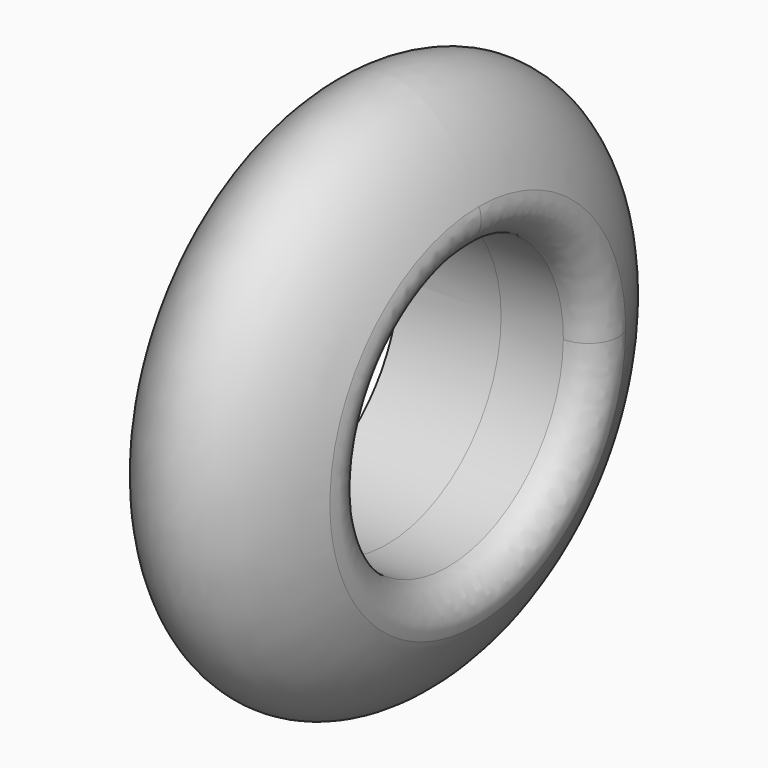
from build123d import *

# Parameters (mm, degrees)
F2_R     = 23.2302893252
F3_DEPTH = 18.4935515739
F4_R     = 20
F5_DEPTH = 18.8526750544
F6_R     = 5
F7_DEPTH = 17.3718996871


with BuildPart() as f1:
    # F0 (on Front) → F1 (revolve)
    with BuildSketch(Plane.XZ):
        with BuildLine():
            Line((-17.606544705, -0.1475060738), (17.5061281593, -0.703891208))
            add(Edge.make_bspline(
                [(17.5061281593, -0.703891208), (25.7537951553, 43.7031499409), (0.1598772489, 44.1087036708), (-25.4340406574, 44.5142574008), (-17.606544705, -0.1475060738)],
                knots=[4.3842952705, 4.3842952705, 4.3842952705, 6.2745397051, 6.2745397051, 8.1647841398, 8.1647841398, 8.1647841398], degree=2, weights=[1, 0.5856438179, 1, 0.5856438179, 1]))
        make_face()
    revolve(axis=Axis((-0.0502082729, 0, -0.4256986409), (0.9998744804, 0, -0.0158437183)))

    # F2 (on Right) → F3 (cut, through all)
    with BuildSketch(Plane.YZ):
        Circle(F2_R)
    extrude(amount=F3_DEPTH, mode=Mode.SUBTRACT)

    # F4 (on Right) → F5 (cut, through all)
    with BuildSketch(Plane.YZ):
        Circle(F4_R)
    extrude(amount=-F5_DEPTH, mode=Mode.SUBTRACT)

    # F6
    f6_edges = [f1.edges().sort_by_distance(p)[0] for p in [
        (17.015314, 16.426459, 16.426131),
        (16.71995, -16.426452, -16.426138),
        (-18.281735, -14.142642, -14.141629),
        (-17.804602, 14.142639, 14.141632),
    ]]
    fillet(f6_edges, radius=F6_R)

    # F7 (cut, through all): a face of the model
    f7_faces = [f1.faces().sort_by_distance(p)[0] for p in [
        (0, -22.5732375208, 0),
    ]]
    extrude(f7_faces, amount=-F7_DEPTH, mode=Mode.SUBTRACT)


solid = f1.part
